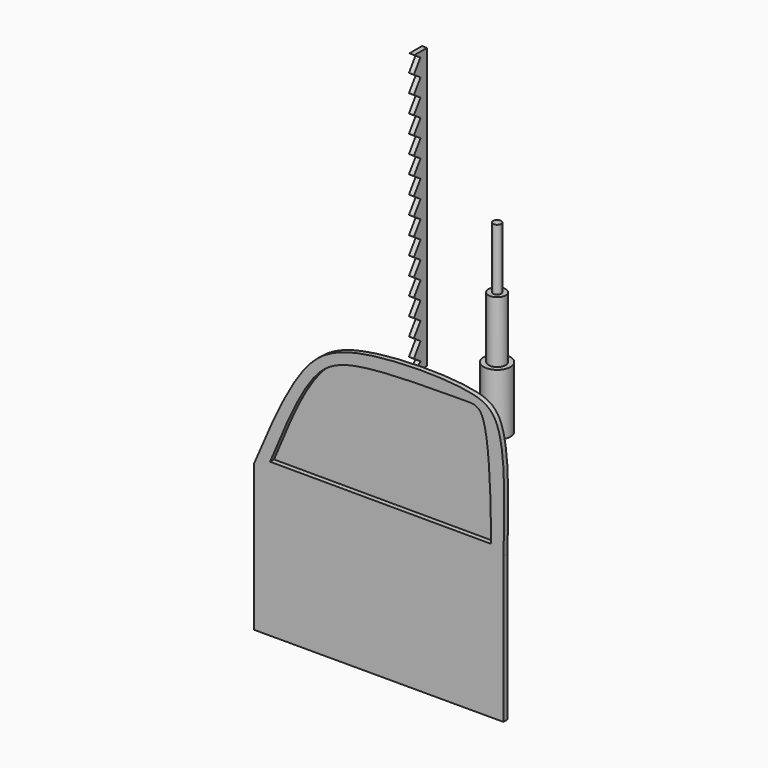
from build123d import *

# Parameters (mm, degrees)
F1_DEPTH  = 2
F3_DEPTH  = 1
F5_DEPTH  = 20
F6_R      = 0.6740837688
F6_R_2    = 0.6794872763
F7_DEPTH  = 2
F8_R      = 1.1503813394
F8_R_2    = 1.1532026448
F9_DEPTH  = 1
F14_W     = 3.547757864
F14_H     = 3.547757864
F15_DEPTH = 110
F16_DEPTH = 4
F17_R     = 5.4389816306
F18_DEPTH = 25
F19_R     = 3.4800068769
F20_DEPTH = 25
F21_R     = 1.6574043711
F22_DEPTH = 25
F25_DEPTH = 25
F27_DEPTH = 2


# Not quite as in the source:
# - a feature names something its author has since deleted; it is built from what else it names


with BuildPart() as f1:
    # F0 (on Front) → F1 (new body)
    with BuildSketch(Plane.XZ):
        with BuildLine():
            Line((-72.9369357123, -81.3669546917), (28.6214776443, -81.3669546917))
            Line((28.6214776443, -81.3669546917), (28.6214776443, -22.0463353619))
            add(Edge.make_bspline(
                [(-72.9369357123, -22.0463353619), (-66.3079296953, -6.3903379982), (-54.8236810491, 20.7324864598), (-33.1368908634, 33.9886563081), (14.1885215953, 34.4693387216), (29.9138992328, 26.3054952003), (29.1285218253, -3.0768949366), (28.6214776443, -22.0463353619)],
                knots=[0, 0, 0, 0, 0.2327586614, 0.4032366747, 0.6349341911, 0.7643114096, 1, 1, 1, 1], degree=3))
            Line((-72.9369357123, -22.0463353619), (-72.9369357123, -81.3669546917))
        make_face()
        with BuildLine():
            Line((23.5529407965, -19.2304815576), (-66.3079296953, -19.0427604541))
            add(Edge.make_bspline(
                [(-66.3079296953, -19.0427604541), (-60.6025988038, -5.2091205775), (-50.8417035049, 18.4579923395), (-32.9418385651, 29.0509048337), (11.2998233245, 28.2534036027), (23.8422582571, 29.4620440208), (23.5609324216, -16.9963213799), (23.5529407965, -19.2304815576)],
                knots=[0, 0, 0, 0, 0.2292277789, 0.3921715308, 0.6301185848, 0.7440435368, 0.9842506716, 0.9842506716, 0.9842506716, 0.9842506716], degree=3))
        make_face(mode=Mode.SUBTRACT)
    extrude(amount=F1_DEPTH)


with BuildPart() as f3:
    # F2 (on face) → F3 (new body)
    with BuildSketch(Plane(origin=(0, 0, 0), x_dir=(-1, 0, 0), z_dir=(0, 1, 0))):
        with BuildLine():
            Line((-23.5529407964, -19.2304815668), (66.3079296953, -19.0427604541))
            add(Edge.make_bspline(
                [(-23.5529407964, -19.2304815668), (-23.269595086, -5.9334404727), (-22.8404862365, 14.5885042855), (-20.184558271, 26.8697861091), (-13.9924322403, 30.0265202781), (31.2151711749, 28.02875343), (44.8400626895, 22.8259909303), (55.9527219343, 6.1579662544), (63.45297845, -12.1512318258), (65.5205113196, -17.1808483014), (66.3079296953, -19.0427604541)],
                knots=[0, 0, 0, 0, 0.1767993283, 0.2727640909, 0.3442462663, 0.5417821056, 0.6587934226, 0.788359659, 0.9213359844, 1, 1, 1, 1], degree=3))
        make_face()
    extrude(amount=F3_DEPTH)


with BuildPart() as f5:
    # F4 (on Right) → F5 (new body, symmetric)
    with BuildSketch(Plane.YZ):
        Polygon((-1.0896978201, -57.8757636249), (-1.0896978201, -72.45323807), (-0.2179905568, -72.45323807), (-0.2179905568, -61.9055777788), (1.2627355754, -61.9055777788), (1.2627355754, -72.45323807), (2.0484484266, -72.45323807), (2.0484484266, -57.8757636249), (0.8171472582, -57.8757636249), (0.8171472582, -59.2663548887), (1.4305444201, -59.2663548887), (1.4305444201, -60.084220022), (-0.5459576496, -60.084220022), (-0.5459576496, -59.2663548887), (0, -59.2663548887), (0, -57.8757636249), align=None)
    extrude(amount=F5_DEPTH, both=True)

    # F6 (on face) → F7 (join)
    with BuildSketch(Plane(origin=(0, 2.0484484266, 0), x_dir=(-1, 0, 0), z_dir=(0, 1, 0))):
        with Locations((-10.6959426776, -67.096978426)):
            Circle(F6_R)
        with Locations((10.5811031535, -67.096978426)):
            Circle(F6_R_2)
    extrude(amount=F7_DEPTH)

    # F8 (on face) → F9 (join)
    with BuildSketch(Plane(origin=(0, 4.0484484266, 0), x_dir=(-1, 0, 0), z_dir=(0, 1, 0))):
        with Locations((-10.6959426776, -67.096978426)):
            Circle(F8_R)
        with Locations((10.6070199981, -67.0710653067)):
            Circle(F8_R_2)
    extrude(amount=F9_DEPTH)


with BuildPart() as f11:
    # F10 (on Right) → F11 (revolve)
    with BuildSketch(Plane.YZ):
        with BuildLine():
            Line((2.1344509079, -62.3869039118), (2.0657987334, -62.3869039118))
            Line((2.0657987334, -62.3869039118), (2.0657987334, -67.175835371))
            Line((2.0657987334, -67.175835371), (3.6893903743, -67.175835371))
            Line((3.6893903743, -67.175835371), (3.6893903743, -63.812112902))
            ThreePointArc((3.6893903743, -63.812112902), (3.0686592581, -62.9285025663), (2.1344509079, -62.3869039118))
        make_face()
    revolve(axis=Axis((0, 4.3976157904, -67.175835371), (0, 1, 0)))

    # F12 (on Right) → F13 (revolve)
    with BuildSketch(Plane.YZ):
        with BuildLine():
            Line((3.290206524, -67.100353539), (5.9968891046, -67.100353539))
            ThreePointArc((5.9968891046, -67.100353539), (4.6435478143, -65.7470122487), (3.290206524, -67.100353539))
        make_face()
    revolve(axis=Axis((0, 4.8515796661, -67.100353539), (0, 1, 0)))


with BuildPart() as f15:
    # F14 (on Top) → F15 (new body)
    with BuildSketch(Plane.XY):
        with Locations((-46.1208410561, 48.1243357062)):
            Rectangle(F14_W, F14_H)
    extrude(amount=F15_DEPTH)

    # F14 (on Top) → F25 (join)
    with BuildSketch(Plane.XY):
        with Locations((-46.1208410561, 48.1243357062)):
            Rectangle(F14_W, F14_H)
    extrude(amount=F25_DEPTH)


with BuildPart() as f16:
    # F4 (on Right) → F16 (new body, symmetric)
    with BuildSketch(Plane.YZ):
        Polygon((0, -45.9536090493), (0, -57.8757636249), (0, -59.2663548887), (-0.5459576496, -59.2663548887), (-0.5459576496, -60.084220022), (1.4305444201, -60.084220022), (1.4305444201, -59.2663548887), (0.8171472582, -59.2663548887), (0.8171472582, -57.8757636249), (0.8171472582, -45.9536090493), align=None)
    extrude(amount=F16_DEPTH, both=True)


with BuildPart() as f18:
    # F17 (on Top) → F18 (new body)
    with BuildSketch(Plane.XY):
        with Locations((0, 30.5617935956)):
            Circle(F17_R)
    extrude(amount=F18_DEPTH)

    # F19 (on face) → F20 (join)
    with BuildSketch(Plane.XY.offset(25)):
        with Locations((0, 30.5617935956)):
            Circle(F19_R)
    extrude(amount=F20_DEPTH)

    # F21 (on face) → F22 (join)
    with BuildSketch(Plane.XY.offset(50)):
        with Locations((0, 30.5617935956)):
            Circle(F21_R)
    extrude(amount=F22_DEPTH)


with BuildPart() as f24:
    # F23 (on Right) → F24 (revolve)
    with BuildSketch(Plane.YZ):
        with BuildLine():
            ThreePointArc((4.4042146765, -51.6518875957), (3.7994878367, -51.0471607558), (3.1947609968, -51.6518875957))
            Line((3.1947609968, -51.6518875957), (4.4042146765, -51.6518875957))
        make_face()
    revolve(axis=Axis((0, 2.626526315, -51.6518875957), (0, 1, 0)))


with BuildPart() as f24b:
    # F23 (on Right) → F24, piece 2 (revolve)
    with BuildSketch(Plane.YZ):
        with BuildLine():
            ThreePointArc((3.1947609968, -49.3592881282), (2.2212167521, -48.3185221094), (0.8488379535, -47.9343883626))
            Line((0.8488379535, -47.9343883626), (0.8488379535, -51.6518875957))
            Line((0.8488379535, -51.6518875957), (3.1947609968, -51.6518875957))
            Line((3.1947609968, -51.6518875957), (3.1947609968, -49.3592881282))
        make_face()
    revolve(axis=Axis((0, 2.626526315, -51.6518875957), (0, 1, 0)))


with BuildPart() as f27:
    # F26 (on face) → F27 (new body)
    with BuildSketch(Plane(origin=(-47.8947199881, 0, 0), x_dir=(0, -1, 0), z_dir=(-1, 0, 0))):
        Polygon((-51.4049215033, 110), (-48.3524078404, 112.1028363705), (-54.7136217356, 112.1028363705), (-54.7136217356, -1.8382943235), (-48.0950288475, -1.8382943235), (-51.4891035855, 1.1467365548), (-48.0950288475, 3.4848698415), (-51.4891035855, 8.4117674623), (-48.0950288475, 10.749900749), (-51.4891035855, 15.6767983698), (-48.0950288475, 18.0149316565), (-51.4891035855, 22.9418292773), (-48.0950288475, 25.279962564), (-51.4891035855, 30.2068601848), (-48.0950288475, 32.5449934715), (-51.4891035855, 37.4718910923), (-48.0950288475, 39.810024379), (-51.4891035855, 44.7369219998), (-48.0950288475, 47.0750552865), (-51.4891035855, 52.0019529073), (-48.0950288475, 54.3400861939), (-51.4891035855, 59.2669838148), (-48.0950288475, 61.6051171014), (-51.4891035855, 66.5320147222), (-48.0950288475, 68.8701480089), (-51.4891035855, 73.7970456297), (-48.0950288475, 76.1351789164), (-51.4891035855, 81.0620765372), (-48.0950288475, 83.4002098239), (-51.4891035855, 88.3271074447), (-48.0950288475, 90.6652407314), (-51.4891035855, 95.5921383522), (-48.0950288475, 97.9302716389), (-51.4891035855, 102.8571692597), (-48.0950288475, 105.1953025464), align=None)
    extrude(amount=F27_DEPTH)


solid = Compound([f1.part, f3.part, f5.part, f11.part, f16.part, f18.part, f24.part, f24b.part, f27.part])
